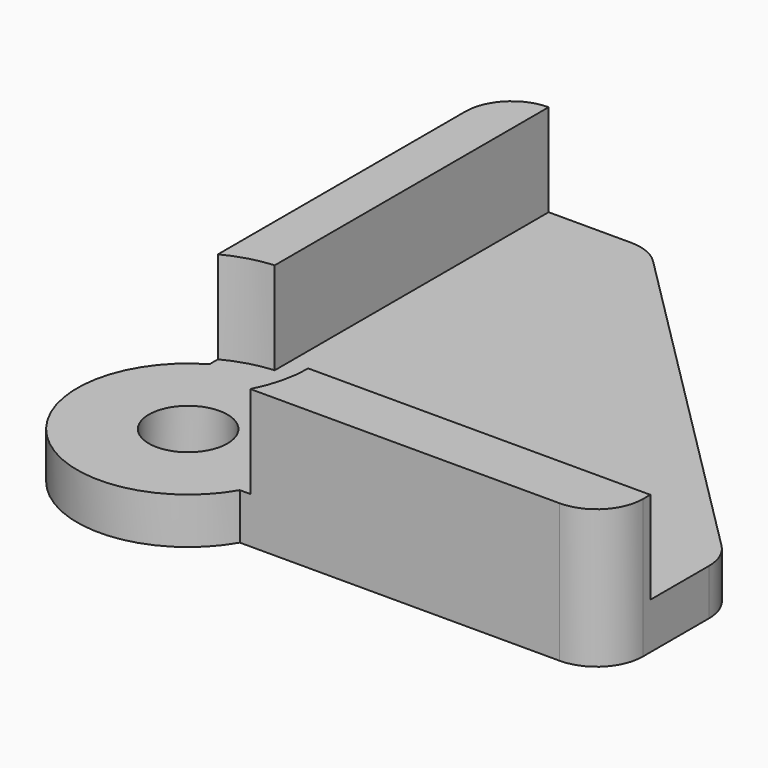
from build123d import *

# Parameters (mm, degrees)
F1_R     = 4.25
F2_DEPTH = 5
F3_DEPTH = 15
F4_R     = 4.99999


# Not quite as in the source:
# - a fillet or chamfer is up to 0.001 mm smaller than in the source, because OpenCascade refuses the exact size
# - a feature names something its author has since deleted; it is built from what else it names


with BuildPart() as f2:
    # F1 (on Top) → F2 (new body)
    with BuildSketch(Plane.XY):
        with BuildLine():
            Line((39.3818591636, 0.8618591636), (-0.6181408364, 0.8618591636))
            Line((-0.6181408364, 0.8618591636), (-0.6181408364, 40.8618591636))
            Line((-0.6181408364, 40.8618591636), (-11.6181408364, 40.8618591636))
            Line((-11.6181408364, 40.8618591636), (-11.6181408364, 3.8233405604))
            ThreePointArc((-11.6181408364, 3.8233405604), (-14.1903183566, 3.3614410672), (-16.6181408364, 2.3944217582))
            Line((-16.6181408364, 2.3944217582), (-16.6181408364, 1.254164009))
            ThreePointArc((-16.6181408364, 1.254164009), (-19.1034222107, -17.6234222107), (-0.225835991, -15.1381408364))
            Line((-0.225835991, -15.1381408364), (0.9144217582, -15.1381408364))
            ThreePointArc((0.9144217582, -15.1381408364), (2.0096719934, -12.2265616521), (2.3818591636, -9.1381408364))
            Line((2.3818591636, -9.1381408364), (39.3818591636, -9.1381408364))
            Line((39.3818591636, -9.1381408364), (39.3818591636, 0.8618591636))
        make_face()
        with Locations((-10.6181408364, -9.1381408364)):
            Circle(F1_R, mode=Mode.SUBTRACT)
        Polygon((-0.6181408364, 40.8618591636), (-0.6181408364, 0.8618591636), (39.3818591636, 0.8618591636), align=None)
    extrude(amount=F2_DEPTH)

    # F1 (on Top) → F3 (join)
    with BuildSketch(Plane.XY):
        with BuildLine():
            Line((39.3818591636, -15.1381408364), (39.3818591636, -9.1381408364))
            Line((39.3818591636, -9.1381408364), (2.3818591636, -9.1381408364))
            ThreePointArc((2.3818591636, -9.1381408364), (2.0096719934, -12.2265616521), (0.9144217582, -15.1381408364))
            Line((0.9144217582, -15.1381408364), (39.3818591636, -15.1381408364))
        make_face()
        with BuildLine():
            Line((-11.6181408364, 3.8233405604), (-11.6181408364, 40.8618591636))
            Line((-11.6181408364, 40.8618591636), (-16.6181408364, 40.8618591636))
            Line((-16.6181408364, 40.8618591636), (-16.6181408364, 2.3944217582))
            ThreePointArc((-16.6181408364, 2.3944217582), (-14.1903183566, 3.3614410672), (-11.6181408364, 3.8233405604))
        make_face()
    extrude(amount=F3_DEPTH)

    # F4 (radius 5 in the source; OpenCascade refuses exactly that, so slightly less here)
    f4_edges = [f2.edges().sort_by_distance(p)[0] for p in [
        (39.381859, -15.138141, 7.5),
        (-16.618141, 40.861859, 7.5),
        (39.381859, 0.861859, 2.5),
        (-0.618141, 40.861859, 2.5),
    ]]
    fillet(f4_edges, radius=F4_R)


solid = f2.part
